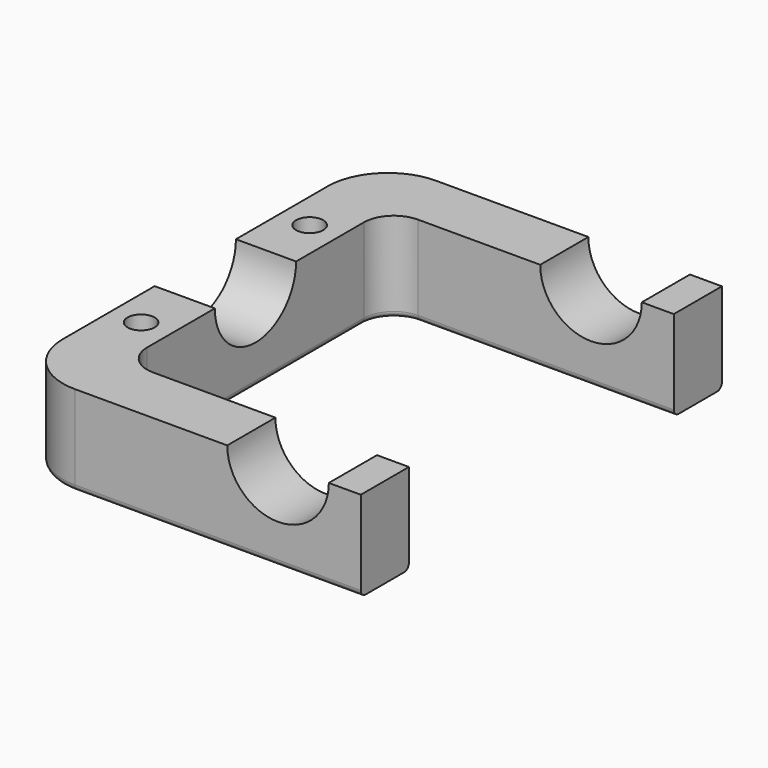
from build123d import *

# Parameters (mm, degrees)
F0_W      = 60
F0_H      = 60
F0_W_2    = 44
F0_H_2    = 44
F1_DEPTH  = 12
F3_DEPTH  = 25
F4_R      = 8
F5_R      = 4
F7_DEPTH  = 25
F9_DEPTH  = 60.001
F10_R     = 1.8
F11_DEPTH = 25
F12_R     = 0.8
F13_R     = 1.8
F14_DEPTH = 2


# Not quite as in the source:
# - a feature names something its author has since deleted; it is built from what else it names


with BuildPart() as f1:
    # F0 (on Top) → F1 (new body)
    with BuildSketch(Plane.XY):
        Rectangle(F0_W, F0_H)
        Rectangle(F0_W_2, F0_H_2, mode=Mode.SUBTRACT)
    extrude(amount=F1_DEPTH)

    # F2 (on face) → F3 (cut)
    with BuildSketch(Plane.XY.offset(12)):
        Polygon((30, -30), (30, 30), (16, 30), (16, 22), (22, 22), (22, -22), (16, -22), (16, -30), align=None)
    extrude(amount=-F3_DEPTH, mode=Mode.SUBTRACT)

    # F4
    f4_edges = [f1.edges().sort_by_distance(p)[0] for p in [
        (-30, -30, 6),
        (-30, 30, 6),
    ]]
    fillet(f4_edges, radius=F4_R)

    # F5
    f5_edges = [f1.edges().sort_by_distance(p)[0] for p in [
        (-22, 22, 6),
        (-22, -22, 6),
    ]]
    fillet(f5_edges, radius=F5_R)

    # F6 (on face) → F7 (cut)
    with BuildSketch(Plane.YZ.offset(-22)):
        with BuildLine():
            ThreePointArc((-6.75, 12), (0, 5.25), (6.75, 12))
            Line((6.75, 12), (-6.75, 12))
        make_face()
    extrude(amount=-F7_DEPTH, mode=Mode.SUBTRACT)

    # F8 (on face) → F9 (cut, through all)
    with BuildSketch(Plane.XZ.offset(30)):
        with BuildLine():
            ThreePointArc((-1.75, 12), (5, 5.25), (11.75, 12))
            Line((11.75, 12), (-1.75, 12))
        make_face()
    extrude(amount=-F9_DEPTH, mode=Mode.SUBTRACT)

    # F10 (on face) → F11 (cut)
    with BuildSketch(Plane.XY.offset(12)):
        with Locations((-26, 14)):
            Circle(F10_R)
        with Locations((-26, -14)):
            Circle(F10_R)
    extrude(amount=-F11_DEPTH, mode=Mode.SUBTRACT)

    # F12
    f12_edges = [f1.edges().sort_by_distance(p)[0] for p in [
        (-3, -30, 0),
        (-20.828427, 20.828427, 0),
    ]]
    fillet(f12_edges, radius=F12_R)

    # F13 (on face) → F14 (cut)
    with BuildSketch(Plane(origin=(0, 0, 0), x_dir=(1, 0, 0), z_dir=(0, 0, -1))):
        Polygon((-23, 12.2679491924), (-23, 15.7320508076), (-26, 17.4641016151), (-29, 15.7320508076), (-29, 12.2679491924), (-26, 10.5358983849), align=None)
        with Locations((-26, 14)):
            Circle(F13_R, mode=Mode.SUBTRACT)
        Polygon((-26, -17.4641016151), (-23, -15.7320508076), (-23, -12.2679491924), (-26, -10.5358983849), (-29, -12.2679491924), (-29, -15.7320508076), align=None)
        with Locations((-26, -14)):
            Circle(F13_R, mode=Mode.SUBTRACT)
    extrude(amount=-F14_DEPTH, mode=Mode.SUBTRACT)


solid = f1.part
